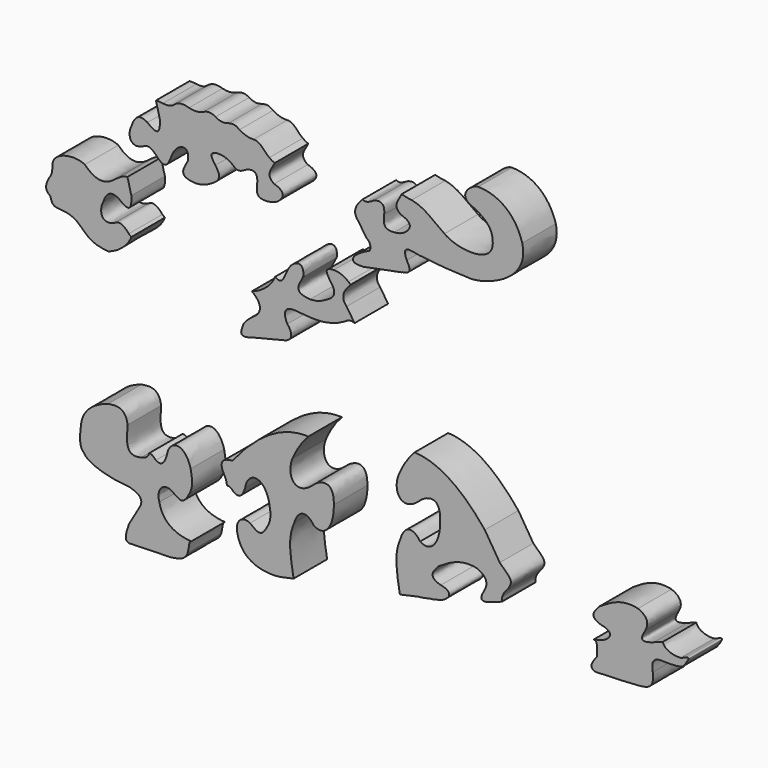
from build123d import *

# Parameters (mm, degrees)
F1_DEPTH = 12
F2_DEPTH = 12


# Not quite as in the source:
# - ends of sketch curves that miss each other by under 0.0002 mm in the source are joined


with BuildPart() as f1:
    # F0 (on Front) → F1 (new body)
    with BuildSketch(Plane.XZ):
        with BuildLine():
            add(Edge.make_bspline(
                [(-57.6632552731, -27.8370372235), (-56.8270192731, -27.7124932235), (-56.4328532731, -28.3077192235), (-55.7004402731, -28.9646112235)],
                knots=[0, 0, 0, 0, 1, 1, 1, 1], degree=3))
            add(Edge.make_bspline(
                [(-59.9392842731, -29.6536852235), (-58.5150639656, -29.3227779134), (-57.7620552726, -28.7312774051), (-57.6632552731, -27.8370372235)],
                knots=[0, 0, 0, 0, 0.574929609, 0.574929609, 0.574929609, 0.574929609], degree=3))
            add(Edge.make_bspline(
                [(-63.8231502731, -22.7211922235), (-63.9633372731, -26.5746232235), (-64.8168222731, -30.7897702235), (-59.9392842731, -29.6536852235)],
                knots=[0, 0, 0, 0, 1, 1, 1, 1], degree=3))
            add(Edge.make_bspline(
                [(-69.4192572731, -19.2131872235), (-67.9895642731, -18.9941012235), (-64.3453622731, -18.0729412235), (-63.8231502731, -22.7211922235)],
                knots=[0, 0, 0, 0, 1, 1, 1, 1], degree=3))
            add(Edge.make_bspline(
                [(-77.1869882731, -27.3985372235), (-76.9230312731, -23.4790862235), (-74.2488692731, -20.7941312235), (-69.4192572731, -19.2131872235)],
                knots=[0, 0, 0, 0, 1, 1, 1, 1], degree=3))
            add(Edge.make_bspline(
                [(-76.3099872731, -33.7881222235), (-77.6117482731, -32.8695732235), (-77.5381322731, -30.3005722235), (-77.1869882731, -27.3985372235)],
                knots=[0, 0, 0, 0, 1, 1, 1, 1], degree=3))
            add(Edge.make_bspline(
                [(-63.3637672731, -38.1313692235), (-70.7173222731, -37.7332332235), (-75.6068892731, -35.4201732235), (-76.3099872731, -33.7881222235)],
                knots=[0, 0, 0, 0, 1, 1, 1, 1], degree=3))
            add(Edge.make_bspline(
                [(-60.2316182731, -42.0569992235), (-58.8391352731, -39.2936542235), (-62.0487202731, -38.5416922235), (-63.3637672731, -38.1313692235)],
                knots=[0, 0, 0, 0, 1, 1, 1, 1], degree=3))
            Line((-60.2316182731, -42.0569992235), (-63.4055302731, -47.5278202235))
            add(Edge.make_bspline(
                [(-62.5285282731, -52.3304492235), (-65.2092132731, -52.7646142235), (-64.2890662731, -50.1306202235), (-63.4055302731, -47.5278202235)],
                knots=[0, 0, 0, 0, 1, 1, 1, 1], degree=3))
            Line((-62.5285282731, -52.3304492235), (-51.5033612731, -52.0381152235))
            add(Edge.make_bspline(
                [(-46.6172052731, -49.3653462235), (-47.5033612731, -51.7611842235), (-49.6774822731, -51.7306562235), (-51.5033612731, -52.0381152235)],
                knots=[0, 0, 0, 0, 1, 1, 1, 1], degree=3))
            add(Edge.make_bspline(
                [(-45.5744562731, -46.1050362235), (-46.3868670531, -46.3715316602), (-46.0201860134, -47.0933507408), (-46.6172052731, -49.3653462235)],
                knots=[0.3924968872, 0.3924968872, 0.3924968872, 0.3924968872, 1, 1, 1, 1], degree=3))
            add(Edge.make_bspline(
                [(-54.7190352731, -39.1963012235), (-53.7864772731, -43.8191412235), (-50.1763782731, -45.8004342235), (-45.5744562731, -46.1050362235)],
                knots=[0, 0, 0, 0, 1, 1, 1, 1], degree=3))
            add(Edge.make_bspline(
                [(-51.1901452731, -35.1662692235), (-53.7689652731, -33.8076662235), (-55.6370502731, -36.2625362235), (-54.7190352731, -39.1963012235)],
                knots=[0, 0, 0, 0, 1, 1, 1, 1], degree=3))
            add(Edge.make_bspline(
                [(-46.0534192731, -34.1222192235), (-47.9555772731, -37.9892172235), (-49.0004562731, -36.7478712235), (-51.1901452731, -35.1662692235)],
                knots=[0, 0, 0, 0, 1, 1, 1, 1], degree=3))
            add(Edge.make_bspline(
                [(-45.7610872731, -27.8788012235), (-45.3743582731, -29.9115232235), (-44.9107912731, -31.9365612235), (-46.0534192731, -34.1222192235)],
                knots=[0, 0, 0, 0, 1, 1, 1, 1], degree=3))
            add(Edge.make_bspline(
                [(-52.5682902731, -26.7094642235), (-51.8971942731, -22.2386062235), (-47.3982782731, -21.8283962235), (-45.7610872731, -27.8788012235)],
                knots=[0, 0, 0, 0, 1, 1, 1, 1], degree=3))
            add(Edge.make_bspline(
                [(-55.7004402731, -28.9646112235), (-53.8401442731, -30.1369062235), (-53.0759262731, -28.2868492235), (-52.5682902731, -26.7094642235)],
                knots=[0, 0, 0, 0, 1, 1, 1, 1], degree=3))
        make_face()
    extrude(amount=F1_DEPTH)


with BuildPart() as f1b:
    # F0 (on Front) → F1, piece 2 (new body)
    with BuildSketch(Plane.XZ):
        with BuildLine():
            add(Edge.make_bspline(
                [(-12.0773014723, -8.7989715469), (-14.2629566343, -11.097880595), (-15.5926600777, -13.4697155345), (-16.6487829582, -15.8648618052)],
                knots=[0.0115110713, 0.0115110713, 0.0115110713, 0.0115110713, 1, 1, 1, 1], degree=3))
            add(Edge.make_bspline(
                [(-33.8134335521, -21.9709454075), (-26.7640223709, -13.1322376429), (-19.5312883541, -8.4546031934), (-12.0773014723, -8.7989715469)],
                knots=[0, 0, 0, 0, 0.5332230593, 0.5332230593, 0.5332230593, 0.5332230593], degree=3))
            add(Edge.make_bspline(
                [(-36.1938665521, -26.1889054075), (-37.7022515521, -23.4593484075), (-36.7586165521, -22.1397024075), (-33.8134335521, -21.9709454075)],
                knots=[0, 0, 0, 0, 1, 1, 1, 1], degree=3))
            add(Edge.make_bspline(
                [(-36.1938665521, -26.1889054075), (-35.2106601216, -27.8341431077), (-35.7371349104, -28.0034519638), (-35.2542215521, -28.7155054075)],
                knots=[0, 0, 0, 0, 2.6956706561, 2.6956706561, 2.6956706561, 2.6956706561], degree=3))
            add(Edge.make_bspline(
                [(-35.2542215521, -28.7155054075), (-34.4179855521, -28.5909614075), (-34.0238195521, -29.1861874075), (-33.2914065521, -29.8430794075)],
                knots=[0, 0, 0, 0, 1, 1, 1, 1], degree=3))
            add(Edge.make_bspline(
                [(-33.2914065521, -29.8430794075), (-31.4311105521, -31.0153744075), (-30.6668925521, -29.1653174075), (-30.1592565521, -27.5879324075)],
                knots=[0, 0, 0, 0, 1, 1, 1, 1], degree=3))
            add(Edge.make_bspline(
                [(-30.1592565521, -27.5879324075), (-29.4881605521, -23.1170744075), (-24.9892445521, -22.7068644075), (-23.3520535521, -28.7572694075)],
                knots=[0, 0, 0, 0, 1, 1, 1, 1], degree=3))
            add(Edge.make_bspline(
                [(-23.3520535521, -28.7572694075), (-22.9653245521, -30.7899914075), (-22.5017575521, -32.8150294075), (-23.6443855521, -35.0006874075)],
                knots=[0, 0, 0, 0, 1, 1, 1, 1], degree=3))
            add(Edge.make_bspline(
                [(-23.6443855521, -35.0006874075), (-25.5465435521, -38.8676854075), (-26.5914225521, -37.6263394075), (-28.7811115521, -36.0447374075)],
                knots=[0, 0, 0, 0, 1, 1, 1, 1], degree=3))
            add(Edge.make_bspline(
                [(-28.7811115521, -36.0447374075), (-31.3599315521, -34.6861344075), (-33.2280165521, -37.1410044075), (-32.3100015521, -40.0747694075)],
                knots=[0, 0, 0, 0, 1, 1, 1, 1], degree=3))
            add(Edge.make_bspline(
                [(-32.3100015521, -40.0747694075), (-31.3655626309, -44.6390467683), (-27.808671917, -46.6098858118), (-23.2706547375, -46.9273209767)],
                knots=[0.0015526306, 0.0015526306, 0.0015526306, 0.0015526306, 0.9912302643, 0.9912302643, 0.9912302643, 0.9912302643], degree=3))
            add(Edge.make_bspline(
                [(-23.2706547375, -46.9273209767), (-23.2304424402, -46.9301338346), (-23.1901531038, -46.9328168656), (-23.1497878636, -46.9353707238)],
                knots=[0.9912302643, 0.9912302643, 0.9912302643, 0.9912302643, 1, 1, 1, 1], degree=3))
            add(Edge.make_bspline(
                [(-23.1497878636, -46.9353707238), (-21.813176476, -47.0200015094), (-20.6810826343, -46.9236295901), (-19.5101269181, -46.6634810166)],
                knots=[0.1098075094, 0.1098075094, 0.1098075094, 0.1098075094, 3.7697720097, 3.7697720097, 3.7697720097, 3.7697720097], degree=3))
            Line((-19.5101269181, -46.6634810166), (-16.2948955521, -45.9731464075))
            add(Edge.make_bspline(
                [(-16.1063455521, -31.8267744075), (-18.2630955521, -36.6973344075), (-17.0116295521, -41.3154354075), (-16.2948955521, -45.9731464075)],
                knots=[0, 0, 0, 0, 1, 1, 1, 1], degree=3))
            add(Edge.make_bspline(
                [(-10.5102365521, -30.7409634075), (-12.7108025521, -27.4498184075), (-15.1357915521, -28.4487944075), (-16.1063455521, -31.8267744075)],
                knots=[0, 0, 0, 0, 1, 1, 1, 1], degree=3))
            add(Edge.make_bspline(
                [(-4.7880627815, -23.6184258893), (-4.6595943077, -28.2050325034), (-6.7065542785, -33.0044090569), (-10.5102365521, -30.7409634075)],
                knots=[0.0038307729, 0.0038307729, 0.0038307729, 0.0038307729, 1, 1, 1, 1], degree=3))
            add(Edge.make_bspline(
                [(-10.2980750893, -20.2109066236), (-9.3285496951, -19.3834559666), (-4.7053523786, -16.6988469177), (-4.7880627815, -23.6184258893)],
                knots=[0, 0, 0, 0, 0.9989651443, 0.9989651443, 0.9989651443, 0.9989651443], degree=3))
            add(Edge.make_bspline(
                [(-16.6487829582, -15.8648618052), (-18.5621299308, -20.733127896), (-15.5459850899, -25.3383312754), (-10.2980750893, -20.2109066236)],
                knots=[0, 0, 0, 0, 0.9983595387, 0.9983595387, 0.9983595387, 0.9983595387], degree=3))
        make_face()
    extrude(amount=F1_DEPTH)


with BuildPart() as f1c:
    # F0 (on Front) → F1, piece 3 (new body)
    with BuildSketch(Plane.XZ):
        with BuildLine():
            add(Edge.make_bspline(
                [(23.548084, -38.2377454075), (22.7367236481, -38.1791038936), (21.4068074297, -38.7869122604), (19.444968, -38.9163794075)],
                knots=[0.5218030141, 0.5218030141, 0.5218030141, 0.5218030141, 1, 1, 1, 1], degree=3))
            add(Edge.make_bspline(
                [(23.548084, -38.2377454075), (24.992613, -37.9112934075), (26.754442, -37.5744944075), (27.651203, -36.5359454075)],
                knots=[0, 0, 0, 0, 1, 1, 1, 1], degree=3))
            add(Edge.make_bspline(
                [(27.651203, -36.5359454075), (29.183317, -35.1405314075), (27.428005, -34.1638224075), (25.813674, -33.9049404075)],
                knots=[0, 0, 0, 0, 1, 1, 1, 1], degree=3))
            add(Edge.make_bspline(
                [(25.813674, -33.9049404075), (22.067411, -32.7916104075), (23.602502, -31.0854724075), (25.187245, -29.3737634075)],
                knots=[0, 0, 0, 0, 1, 1, 1, 1], degree=3))
            add(Edge.make_bspline(
                [(25.187245, -29.3737634075), (28.494805, -27.1301704075), (31.936191, -25.3252374075), (36.233293, -26.3251364075)],
                knots=[0, 0, 0, 0, 1, 1, 1, 1], degree=3))
            add(Edge.make_bspline(
                [(36.233293, -26.3251364075), (38.786761, -27.3891544075), (39.546997, -28.9989354075), (38.258748, -31.2321714075)],
                knots=[0, 0, 0, 0, 1, 1, 1, 1], degree=3))
            add(Edge.make_bspline(
                [(38.258748, -31.2321714075), (37.095832, -33.2535824075), (36.489915, -34.9055584075), (40.701825, -33.3620344075)],
                knots=[0, 0, 0, 0, 1, 1, 1, 1], degree=3))
            Line((40.701825, -33.3620344075), (43.353712, -32.3806264075))
            Line((43.353712, -32.3806264075), (43.332833, -32.0674104075))
            add(Edge.make_bspline(
                [(44.37688, -29.3528814075), (43.463575, -30.5304284075), (43.186687, -31.5743714075), (43.332833, -32.0674104075)],
                knots=[0, 0, 0, 0, 1, 1, 1, 1], degree=3))
            add(Edge.make_bspline(
                [(42.706401, -22.7544864075), (45.116582, -25.3982344075), (47.511246, -25.9690594075), (44.37688, -29.3528814075)],
                knots=[0, 0, 0, 0, 1, 1, 1, 1], degree=3))
            Line((42.706401, -22.7544864075), (38.4217117968, -15.8964642394))
            add(Edge.make_bspline(
                [(18.3372880795, -2.9005945461), (24.854509263, -3.2016850576), (31.5408666488, -7.3418331273), (38.4217117968, -15.8964642394)],
                knots=[0.5332230593, 0.5332230593, 0.5332230593, 0.5332230593, 0.9994343196, 0.9994343196, 0.9994343196, 0.9994343196], degree=3))
            add(Edge.make_bspline(
                [(18.3372880798, -2.9005945469), (16.150032215, -5.2027873429), (14.8206613203, -7.5774711635), (13.765336, -9.9753144075)],
                knots=[0.0107004763, 0.0107004763, 0.0107004763, 0.0107004763, 1, 1, 1, 1], degree=3))
            add(Edge.make_bspline(
                [(13.765336, -9.9753144075), (11.863534, -14.8573274075), (14.90662, -19.4605244075), (20.154924, -14.2768024075)],
                knots=[0, 0, 0, 0, 1, 1, 1, 1], degree=3))
            add(Edge.make_bspline(
                [(20.154924, -14.2768024075), (21.124766, -13.4476894075), (25.754308, -10.7545304075), (25.667508, -17.7012834075)],
                knots=[0, 0, 0, 0, 1, 1, 1, 1], degree=3))
            add(Edge.make_bspline(
                [(25.667508, -17.7012834075), (25.785906, -22.3045624075), (23.709086, -27.1373974075), (19.904353, -24.8425864075)],
                knots=[0, 0, 0, 0, 1, 1, 1, 1], degree=3))
            add(Edge.make_bspline(
                [(19.904353, -24.8425864075), (17.703787, -21.5514414075), (15.278798, -22.5504174075), (14.308244, -25.9283974075)],
                knots=[0, 0, 0, 0, 1, 1, 1, 1], degree=3))
            add(Edge.make_bspline(
                [(14.308244, -25.9283974075), (12.151494, -30.7989574075), (13.40296, -35.4170584075), (14.119694, -40.0747694075)],
                knots=[0, 0, 0, 0, 1, 1, 1, 1], degree=3))
            Line((14.119694, -40.0747694075), (19.444968, -38.9163794075))
        make_face()
    extrude(amount=F1_DEPTH)


with BuildPart() as f1d:
    # F0 (on Front) → F1, piece 4 (new body)
    with BuildSketch(Plane.XZ):
        with BuildLine():
            add(Edge.make_bspline(
                [(69.5825900088, -33.375106762), (71.0271190088, -33.048654762), (72.7889480088, -32.711855762), (73.6857090088, -31.673306762)],
                knots=[0, 0, 0, 0, 1, 1, 1, 1], degree=3))
            add(Edge.make_bspline(
                [(70.5326770088, -37.436461762), (70.7388854588, -34.2937310778), (70.470917436, -33.4379439087), (69.5825900088, -33.375106762)],
                knots=[0, 0, 0, 0, 0.5225537589, 0.5225537589, 0.5225537589, 0.5225537589], degree=3))
            add(Edge.make_bspline(
                [(70.1985800088, -41.362091762), (67.8998800088, -40.913027762), (69.2521470088, -38.938115762), (70.5326770088, -37.436461762)],
                knots=[0, 0, 0, 0, 1, 1, 1, 1], degree=3))
            add(Edge.make_bspline(
                [(82.7271800088, -40.777422762), (76.0265000088, -41.297747762), (73.0870540088, -41.188363762), (70.1985800088, -41.362091762)],
                knots=[0, 0, 0, 0, 1, 1, 1, 1], degree=3))
            add(Edge.make_bspline(
                [(86.4857600088, -36.100077762), (87.0471980088, -40.271784762), (84.8822210088, -40.517448762), (82.7271800088, -40.777422762)],
                knots=[0, 0, 0, 0, 1, 1, 1, 1], degree=3))
            add(Edge.make_bspline(
                [(90.1608150088, -32.425022762), (86.0196750088, -32.014168762), (86.1514170088, -34.000296762), (86.4857600088, -36.100077762)],
                knots=[0, 0, 0, 0, 1, 1, 1, 1], degree=3))
            add(Edge.make_bspline(
                [(95.2557780088, -31.715069762), (94.4564490088, -32.435261762), (91.8822600088, -32.422067762), (90.1608150088, -32.425022762)],
                knots=[0, 0, 0, 0, 1, 1, 1, 1], degree=3))
            add(Edge.make_bspline(
                [(94.4205390088, -29.919303762), (95.4349870088, -29.763903762), (98.4317210088, -27.577872762), (95.2557780088, -31.715069762)],
                knots=[0, 0, 0, 0, 1, 1, 1, 1], degree=3))
            add(Edge.make_bspline(
                [(89.3882180088, -27.517987762), (89.6266837425, -29.1229862778), (92.2412113727, -30.0924736633), (94.4205390088, -29.919303762)],
                knots=[0.061437137, 0.061437137, 0.061437137, 0.061437137, 1, 1, 1, 1], degree=3))
            Line((89.3882180088, -27.517987762), (86.7363310088, -28.499395762))
            add(Edge.make_bspline(
                [(84.2932540088, -26.369532762), (83.1303380088, -28.390943762), (82.5244210088, -30.042919762), (86.7363310088, -28.499395762)],
                knots=[0, 0, 0, 0, 1, 1, 1, 1], degree=3))
            add(Edge.make_bspline(
                [(82.2677990088, -21.462497762), (84.8212670088, -22.526515762), (85.5815030088, -24.136296762), (84.2932540088, -26.369532762)],
                knots=[0, 0, 0, 0, 1, 1, 1, 1], degree=3))
            add(Edge.make_bspline(
                [(71.2217510088, -24.511124762), (74.5293110088, -22.267531762), (77.9706970088, -20.462598762), (82.2677990088, -21.462497762)],
                knots=[0, 0, 0, 0, 1, 1, 1, 1], degree=3))
            add(Edge.make_bspline(
                [(71.8481800088, -29.042301762), (68.1019170088, -27.928971762), (69.6370080088, -26.222833762), (71.2217510088, -24.511124762)],
                knots=[0, 0, 0, 0, 1, 1, 1, 1], degree=3))
            add(Edge.make_bspline(
                [(73.6857090088, -31.673306762), (75.2178230088, -30.277892762), (73.4625110088, -29.301183762), (71.8481800088, -29.042301762)],
                knots=[0, 0, 0, 0, 1, 1, 1, 1], degree=3))
        make_face()
    extrude(amount=F1_DEPTH)


with BuildPart() as f2:
    # F0 (on Front) → F2 (new body)
    with BuildSketch(Plane.XZ):
        with BuildLine():
            add(Edge.make_bspline(
                [(-69.3341766052, 19.2094726506), (-74.1750692719, 19.6497229208), (-75.1314553584, 21.0380042156), (-77.6239506052, 23.3082766506)],
                knots=[0.0007320493, 0.0007320493, 0.0007320493, 0.0007320493, 1, 1, 1, 1], degree=3))
            add(Edge.make_bspline(
                [(-69.3341766052, 19.2094726506), (-66.7822206052, 20.0185446506), (-63.8352736052, 22.0949326506), (-62.7357806052, 24.9935096506)],
                knots=[0, 0, 0, 0, 1, 1, 1, 1], degree=3))
            Line((-62.7357806052, 24.9935096506), (-63.4494586052, 25.5821016506))
            add(Edge.make_bspline(
                [(-67.4655646052, 27.0290806506), (-66.3722566052, 27.8827886506), (-65.0438666052, 27.4566046506), (-63.4494586052, 25.5821016506)],
                knots=[0, 0, 0, 0, 1, 1, 1, 1], degree=3))
            add(Edge.make_bspline(
                [(-70.7729466051, 31.2223666506), (-72.1112546052, 28.6972756506), (-71.3180636052, 25.2035596506), (-67.4655646052, 27.0290806506)],
                knots=[0, 0, 0, 0, 1, 1, 1, 1], degree=3))
            add(Edge.make_bspline(
                [(-66.2548266051, 33.4371306506), (-68.6348356051, 34.8837986506), (-69.9636576051, 33.7024986506), (-70.7729466051, 31.2223666506)],
                knots=[0, 0, 0, 0, 1, 1, 1, 1], degree=3))
            add(Edge.make_bspline(
                [(-62.7407346051, 35.4451836506), (-62.4579096051, 30.6639896506), (-64.2978666051, 31.8851406506), (-66.2548266051, 33.4371306506)],
                knots=[0, 0, 0, 0, 1, 1, 1, 1], degree=3))
            Line((-62.7407346052, 35.4451836506), (-63.8424736052, 39.7668176506))
            add(Edge.make_bspline(
                [(-67.2293236052, 38.1619616506), (-66.2370793141, 38.8034373603), (-65.4511063612, 39.6056437767), (-63.8424736052, 39.7668176506)],
                knots=[0, 0, 0, 0, 0.7472132911, 0.7472132911, 0.7472132911, 0.7472132911], degree=3))
            add(Edge.make_bspline(
                [(-76.0588506052, 38.9002166506), (-73.5317016052, 36.4139846506), (-70.7729876052, 35.1746446506), (-67.2293236052, 38.1619616506)],
                knots=[0, 0, 0, 0, 1, 1, 1, 1], degree=3))
            add(Edge.make_bspline(
                [(-85.3018006052, 36.0062576506), (-85.0422796052, 39.4741636506), (-78.7124016052, 40.4346446506), (-76.0588506052, 38.9002166506)],
                knots=[0, 0, 0, 0, 1, 1, 1, 1], degree=3))
            add(Edge.make_bspline(
                [(-86.1877056052, 32.3740446506), (-85.6062626052, 32.9607836506), (-85.2719136052, 34.0863706506), (-85.3018006052, 36.0062576506)],
                knots=[0, 0, 0, 0, 1, 1, 1, 1], degree=3))
            add(Edge.make_bspline(
                [(-85.8628736052, 27.7673336506), (-87.8424026052, 28.9089566506), (-87.1533056052, 30.6123946506), (-86.1877056052, 32.3740446506)],
                knots=[0, 0, 0, 0, 1, 1, 1, 1], degree=3))
            add(Edge.make_bspline(
                [(-83.4118676052, 25.3753876506), (-85.2312576052, 25.3612486506), (-85.6790836052, 26.4574196506), (-85.8628736052, 27.7673336506)],
                knots=[0, 0, 0, 0, 1, 1, 1, 1], degree=3))
            add(Edge.make_bspline(
                [(-77.6239506052, 23.3082766506), (-79.5033466052, 24.9955086506), (-81.4551646052, 25.2343016506), (-83.4118676052, 25.3753876506)],
                knots=[0, 0, 0, 0, 1, 1, 1, 1], degree=3))
        make_face()
    extrude(amount=F2_DEPTH)


with BuildPart() as f2b:
    # F0 (on Front) → F2, piece 2 (new body)
    with BuildSketch(Plane.XZ):
        with BuildLine():
            Line((-55.6936267021, 61.679005653), (-54.5918877021, 57.357371653))
            add(Edge.make_bspline(
                [(-54.5918877021, 57.357371653), (-54.3090627021, 52.576177653), (-56.1490197021, 53.797328653), (-58.1059797021, 55.349318653)],
                knots=[0, 0, 0, 0, 1, 1, 1, 1], degree=3))
            add(Edge.make_bspline(
                [(-58.1059797021, 55.349318653), (-60.4859887021, 56.795986653), (-61.8148107021, 55.614686653), (-62.6240997021, 53.134554653)],
                knots=[0, 0, 0, 0, 1, 1, 1, 1], degree=3))
            add(Edge.make_bspline(
                [(-62.6240997021, 53.134554653), (-63.9624077021, 50.609463653), (-63.1692167021, 47.115747653), (-59.3167177021, 48.941268653)],
                knots=[0, 0, 0, 0, 1, 1, 1, 1], degree=3))
            add(Edge.make_bspline(
                [(-59.3167177021, 48.941268653), (-58.2234097021, 49.794976653), (-56.8950197021, 49.368792653), (-55.3006117021, 47.494289653)],
                knots=[0, 0, 0, 0, 1, 1, 1, 1], degree=3))
            add(Edge.make_bspline(
                [(-55.3006117021, 47.494289653), (-52.2589077021, 44.482743653), (-51.9397537021, 47.963432653), (-50.9301437021, 49.797642653)],
                knots=[0, 0, 0, 0, 1, 1, 1, 1], degree=3))
            add(Edge.make_bspline(
                [(-50.9301437021, 49.797642653), (-49.7324007021, 52.682575653), (-45.9159127021, 53.956382653), (-46.5301467021, 49.502339653)],
                knots=[0, 0, 0, 0, 1, 1, 1, 1], degree=3))
            add(Edge.make_bspline(
                [(-46.5301467021, 49.502339653), (-47.8736427021, 47.033665653), (-49.5123127021, 44.815469653), (-44.5220927021, 44.511739653)],
                knots=[0, 0, 0, 0, 1, 1, 1, 1], degree=3))
            add(Edge.make_bspline(
                [(-44.5220927021, 44.511739653), (-42.2621227021, 44.496838653), (-40.6673497021, 45.403000653), (-39.1180677021, 46.372139653)],
                knots=[0, 0, 0, 0, 1, 1, 1, 1], degree=3))
            add(Edge.make_bspline(
                [(-39.1180677021, 46.372139653), (-36.8576087021, 47.834099653), (-37.5576867021, 49.343810653), (-38.7046437021, 50.860729653)],
                knots=[0, 0, 0, 0, 1, 1, 1, 1], degree=3))
            add(Edge.make_bspline(
                [(-38.7046437021, 50.860729653), (-39.7865937021, 52.463487653), (-40.8362027021, 54.054064653), (-37.7301467021, 54.079520653)],
                knots=[0, 0, 0, 0, 1, 1, 1, 1], degree=3))
            add(Edge.make_bspline(
                [(-37.7301467021, 54.079520653), (-36.4353057021, 54.059909653), (-35.0827527021, 53.722878653), (-33.5663897021, 52.484890653)],
                knots=[0, 0, 0, 0, 1, 1, 1, 1], degree=3))
            add(Edge.make_bspline(
                [(-33.5663897021, 52.484890653), (-32.1514467021, 51.031914653), (-30.9233427021, 52.070152653), (-29.6684077021, 52.750662653)],
                knots=[0, 0, 0, 0, 1, 1, 1, 1], degree=3))
            add(Edge.make_bspline(
                [(-29.6684077021, 52.750662653), (-27.4842107021, 53.532383653), (-26.5052297021, 52.688465653), (-26.7153867021, 50.240595653)],
                knots=[0, 0, 0, 0, 1, 1, 1, 1], degree=3))
            add(Edge.make_bspline(
                [(-26.7153867021, 50.240595653), (-26.6596527021, 48.588823653), (-27.6647707021, 46.399154653), (-23.8804897021, 46.637911653)],
                knots=[0, 0, 0, 0, 1, 1, 1, 1], degree=3))
            add(Edge.make_bspline(
                [(-23.8804897021, 46.637911653), (-22.0209217021, 46.765060653), (-20.9789237021, 47.371841653), (-20.2187437021, 48.143953653)],
                knots=[0, 0, 0, 0, 1, 1, 1, 1], degree=3))
            add(Edge.make_bspline(
                [(-20.2187437021, 48.143953653), (-18.2333017021, 50.109200653), (-20.2277467021, 51.191590653), (-21.8429047021, 51.658045653)],
                knots=[0, 0, 0, 0, 1, 1, 1, 1], degree=3))
            add(Edge.make_bspline(
                [(-21.8429047021, 51.658045653), (-23.4384897021, 52.654926653), (-23.4653657021, 53.838559653), (-22.7288117021, 55.113077653)],
                knots=[0, 0, 0, 0, 1, 1, 1, 1], degree=3))
            Line((-22.7288117021, 55.113077653), (-21.6934617021, 56.973479653))
            add(Edge.make_bspline(
                [(-23.2352727021, 57.856979653), (-22.7594168865, 57.4575588944), (-22.2313131482, 57.1792315199), (-21.6934617021, 56.973479653)],
                knots=[0, 0, 0, 0, 0.3520102972, 0.3520102972, 0.3520102972, 0.3520102972], degree=3))
            add(Edge.make_bspline(
                [(-27.7194147021, 60.960055653), (-25.7063097021, 61.042991653), (-24.8282167021, 58.869741653), (-23.2352727021, 57.856979653)],
                knots=[0, 0, 0, 0, 1, 1, 1, 1], degree=3))
            add(Edge.make_bspline(
                [(-31.8241107021, 62.052672653), (-30.6899077021, 61.532447653), (-29.7527837021, 60.880836653), (-27.7194147021, 60.960055653)],
                knots=[0, 0, 0, 0, 1, 1, 1, 1], degree=3))
            add(Edge.make_bspline(
                [(-34.8657187021, 62.731866653), (-33.9431007021, 62.815724653), (-33.1190787021, 63.234810653), (-31.8241107021, 62.052672653)],
                knots=[0, 0, 0, 0, 1, 1, 1, 1], degree=3))
            add(Edge.make_bspline(
                [(-38.5865247021, 63.115759653), (-37.5006467021, 62.370237653), (-36.2665627021, 62.217533653), (-34.8657187021, 62.731866653)],
                knots=[0, 0, 0, 0, 1, 1, 1, 1], degree=3))
            add(Edge.make_bspline(
                [(-42.0710857021, 63.233879653), (-40.8220077021, 63.894971653), (-39.6785477021, 63.711109653), (-38.5865247021, 63.115759653)],
                knots=[0, 0, 0, 0, 1, 1, 1, 1], degree=3))
            add(Edge.make_bspline(
                [(-46.2643717021, 62.909047653), (-44.8325377021, 62.574369653), (-43.4244627021, 62.548585653), (-42.0710857021, 63.233879653)],
                knots=[0, 0, 0, 0, 1, 1, 1, 1], degree=3))
            add(Edge.make_bspline(
                [(-50.2509497021, 62.525155653), (-49.2369337021, 63.212839653), (-47.9853327021, 63.478150653), (-46.2643717021, 62.909047653)],
                knots=[0, 0, 0, 0, 1, 1, 1, 1], degree=3))
            add(Edge.make_bspline(
                [(-53.7355117021, 61.580189653), (-52.6204677021, 61.500117653), (-51.5183507021, 61.310191653), (-50.2509497021, 62.525155653)],
                knots=[0, 0, 0, 0, 1, 1, 1, 1], degree=3))
            add(Edge.make_bspline(
                [(-55.6936267021, 61.679005653), (-55.1482861317, 61.730756549), (-54.5088903028, 61.7083162192), (-53.7355117021, 61.580189653)],
                knots=[0.7466347862, 0.7466347862, 0.7466347862, 0.7466347862, 1, 1, 1, 1], degree=3))
        make_face()
    extrude(amount=F2_DEPTH)


with BuildPart() as f2c:
    # F0 (on Front) → F2, piece 3 (new body)
    with BuildSketch(Plane.XZ):
        with BuildLine():
            add(Edge.make_bspline(
                [(1.140997, 24.057427), (0.4143117249, 24.4056286712), (-0.6256048198, 24.4537921928), (-1.31001, 23.762124)],
                knots=[0.3358339564, 0.3358339564, 0.3358339564, 0.3358339564, 0.7562493145, 0.7562493145, 0.7562493145, 0.7562493145], degree=3))
            add(Edge.make_bspline(
                [(1.140997, 24.057427), (0.10911, 25.489662), (-0.066584, 26.059833), (-1.132831, 27.512459)],
                knots=[0, 0, 0, 0, 1, 1, 1, 1], degree=3))
            add(Edge.make_bspline(
                [(-1.132831, 27.512459), (-2.46674, 28.924976), (-2.337564, 30.470498), (-1.073771, 32.119168)],
                knots=[0, 0, 0, 0, 1, 1, 1, 1], degree=3))
            Line((-1.073771, 32.119168), (0.048379, 33.418497))
            Line((0.048379, 33.418497), (-0.601285, 33.92051))
            add(Edge.make_bspline(
                [(-4.765042, 35.51514), (-3.470201, 35.495529), (-2.117648, 35.158498), (-0.601285, 33.92051)],
                knots=[0, 0, 0, 0, 1, 1, 1, 1], degree=3))
            add(Edge.make_bspline(
                [(-5.739539, 32.296349), (-6.821489, 33.899107), (-7.871098, 35.489684), (-4.765042, 35.51514)],
                knots=[0, 0, 0, 0, 1, 1, 1, 1], degree=3))
            add(Edge.make_bspline(
                [(-6.152963, 27.807759), (-3.892504, 29.269719), (-4.592582, 30.77943), (-5.739539, 32.296349)],
                knots=[0, 0, 0, 0, 1, 1, 1, 1], degree=3))
            add(Edge.make_bspline(
                [(-11.556988, 25.947359), (-9.297018, 25.932458), (-7.702245, 26.83862), (-6.152963, 27.807759)],
                knots=[0, 0, 0, 0, 1, 1, 1, 1], degree=3))
            add(Edge.make_bspline(
                [(-13.565042, 30.937959), (-14.908538, 28.469285), (-16.547208, 26.251089), (-11.556988, 25.947359)],
                knots=[0, 0, 0, 0, 1, 1, 1, 1], degree=3))
            add(Edge.make_bspline(
                [(-17.9579480355, 31.2268088923), (-16.7685376208, 34.1041335962), (-12.9807226228, 35.3846972885), (-13.565042, 30.937959)],
                knots=[0.0024980002, 0.0024980002, 0.0024980002, 0.0024980002, 1, 1, 1, 1], degree=3))
            add(Edge.make_bspline(
                [(-21.6147380355, 28.3348638923), (-19.3489549287, 26.5944978854), (-18.917449732, 29.5926467395), (-17.9579480355, 31.2268088923)],
                knots=[0.0948966859, 0.0948966859, 0.0948966859, 0.0948966859, 1, 1, 1, 1], degree=3))
            add(Edge.make_bspline(
                [(-28.2131340355, 22.5508268923), (-25.6611780355, 23.3598988923), (-22.7142310355, 25.4362868923), (-21.6147380355, 28.3348638923)],
                knots=[0, 0, 0, 0, 1, 1, 1, 1], degree=3))
            add(Edge.make_bspline(
                [(-26.824096, 17.029241), (-25.2017497424, 18.7885127325), (-25.8208700002, 20.6351262288), (-28.2131340355, 22.5508268923)],
                knots=[0, 0, 0, 0, 0.9999630963, 0.9999630963, 0.9999630963, 0.9999630963], degree=3))
            add(Edge.make_bspline(
                [(-30.603961, 13.603735), (-29.898478, 14.668907), (-28.313218, 16.035308), (-26.824096, 17.029241)],
                knots=[0, 0, 0, 0, 1, 1, 1, 1], degree=3))
            add(Edge.make_bspline(
                [(-28.212015, 10.916491), (-32.489368, 9.450163), (-31.269579, 11.724053), (-30.603961, 13.603735)],
                knots=[0, 0, 0, 0, 1, 1, 1, 1], degree=3))
            Line((-28.212015, 10.916491), (-18.777554, 13.255312))
            add(Edge.make_bspline(
                [(-18.08316, 17.590313), (-16.347829, 15.485903), (-16.73895, 13.78725), (-18.777554, 13.255312)],
                knots=[0, 0, 0, 0, 1, 1, 1, 1], degree=3))
            add(Edge.make_bspline(
                [(-15.1892, 21.69501), (-18.418522, 22.007017), (-19.730985, 20.896834), (-18.08316, 17.590313)],
                knots=[0, 0, 0, 0, 1, 1, 1, 1], degree=3))
            add(Edge.make_bspline(
                [(-1.31001, 23.762124), (-6.403165, 20.687442), (-10.785689, 21.244854), (-15.1892, 21.69501)],
                knots=[0, 0, 0, 0, 1, 1, 1, 1], degree=3))
        make_face()
    extrude(amount=F2_DEPTH)


with BuildPart() as f2d:
    # F0 (on Front) → F2, piece 4 (new body)
    with BuildSketch(Plane.XZ):
        with BuildLine():
            add(Edge.make_bspline(
                [(4.5253321359, 46.6179367231), (3.4934451359, 48.0501717231), (3.3177511359, 48.6203427231), (2.2515041359, 50.0729687231)],
                knots=[0, 0, 0, 0, 1, 1, 1, 1], degree=3))
            add(Edge.make_bspline(
                [(5.0864031359, 43.5172657231), (6.0313272824, 43.707837226), (5.8822401042, 45.9498901621), (4.5253321359, 46.6179367231)],
                knots=[0, 0, 0, 0, 0.6957238542, 0.6957238542, 0.6957238542, 0.6957238542], degree=3))
            add(Edge.make_bspline(
                [(1.1293571359, 41.0072007231), (2.2197231359, 42.0153747231), (3.5506401359, 42.8431377231), (5.0864031359, 43.5172657231)],
                knots=[0, 0, 0, 0, 1, 1, 1, 1], degree=3))
            add(Edge.make_bspline(
                [(3.6575911359, 39.0746357231), (1.2164261359, 38.9444357231), (-0.0140268641, 39.3193957231), (1.1293571359, 41.0072007231)],
                knots=[0, 0, 0, 0, 1, 1, 1, 1], degree=3))
            Line((3.6575911359, 39.0746357231), (14.5411301359, 41.2354057231))
            add(Edge.make_bspline(
                [(16.0960981359, 44.7596327231), (18.0703531359, 41.3189997231), (15.7572541359, 41.7824367231), (14.5411301359, 41.2354057231)],
                knots=[0, 0, 0, 0, 1, 1, 1, 1], degree=3))
            add(Edge.make_bspline(
                [(19.7038491359, 47.1790087231), (17.3362341359, 47.5033127231), (14.3880751359, 48.7373917231), (16.0960981359, 44.7596327231)],
                knots=[0, 0, 0, 0, 1, 1, 1, 1], degree=3))
            add(Edge.make_bspline(
                [(34.6461251359, 46.0568617231), (28.9467601359, 46.1229357231), (24.3276091359, 46.6519617231), (19.7038491359, 47.1790087231)],
                knots=[0, 0, 0, 0, 1, 1, 1, 1], degree=3))
            add(Edge.make_bspline(
                [(49.1454491359, 59.8474617231), (51.3903551359, 50.1800747231), (38.7751741359, 46.2719467231), (34.6461251359, 46.0568617231)],
                knots=[0, 0, 0, 0, 1, 1, 1, 1], degree=3))
            add(Edge.make_bspline(
                [(36.5655861359, 69.9172567231), (41.6036501359, 69.8747787231), (47.0213151359, 66.9937967231), (49.1454491359, 59.8474617231)],
                knots=[0, 0, 0, 0, 1, 1, 1, 1], degree=3))
            add(Edge.make_bspline(
                [(35.6206211359, 64.0998087231), (29.9587811359, 65.8704497231), (34.2366801359, 69.7204067231), (36.5655861359, 69.9172567231)],
                knots=[0, 0, 0, 0, 1, 1, 1, 1], degree=3))
            add(Edge.make_bspline(
                [(40.6702851359, 57.5736367231), (40.6831541359, 60.7384157231), (38.4164271359, 62.5734247231), (35.6206211359, 64.0998087231)],
                knots=[0, 0, 0, 0, 1, 1, 1, 1], degree=3))
            add(Edge.make_bspline(
                [(26.8796851359, 54.9749797231), (30.5509901359, 52.1310147231), (41.3247501359, 51.0854357231), (40.6702851359, 57.5736367231)],
                knots=[0, 0, 0, 0, 1, 1, 1, 1], degree=3))
            add(Edge.make_bspline(
                [(17.5040291359, 60.3942047231), (21.5489111359, 59.5401197231), (23.4462371359, 57.1484067231), (26.8796851359, 54.9749797231)],
                knots=[0, 0, 0, 0, 1, 1, 1, 1], degree=3))
            add(Edge.make_bspline(
                [(14.6559781359, 60.9696087231), (15.6328199859, 60.5993849706), (16.6559649971, 60.5055858935), (17.5040291359, 60.3942047231)],
                knots=[0.2599849916, 0.2599849916, 0.2599849916, 0.2599849916, 0.8890068216, 0.8890068216, 0.8890068216, 0.8890068216], degree=3))
            Line((14.6559781359, 60.9696087231), (13.6206281359, 59.1092067231))
            add(Edge.make_bspline(
                [(14.5065351359, 55.6541747231), (12.9109501359, 56.6510557231), (12.8840741359, 57.8346887231), (13.6206281359, 59.1092067231)],
                knots=[0, 0, 0, 0, 1, 1, 1, 1], degree=3))
            add(Edge.make_bspline(
                [(16.1306961359, 52.1400827231), (18.1161381359, 54.1053297231), (16.1216931359, 55.1877197231), (14.5065351359, 55.6541747231)],
                knots=[0, 0, 0, 0, 1, 1, 1, 1], degree=3))
            add(Edge.make_bspline(
                [(12.4689501359, 50.6340407231), (14.3285181359, 50.7611897231), (15.3705161359, 51.3679707231), (16.1306961359, 52.1400827231)],
                knots=[0, 0, 0, 0, 1, 1, 1, 1], degree=3))
            add(Edge.make_bspline(
                [(9.6340531359, 54.2367247231), (9.6897871359, 52.5849527231), (8.6846691359, 50.3952837231), (12.4689501359, 50.6340407231)],
                knots=[0, 0, 0, 0, 1, 1, 1, 1], degree=3))
            add(Edge.make_bspline(
                [(6.6810321359, 56.7467917231), (8.8652291359, 57.5285127231), (9.8442101359, 56.6845947231), (9.6340531359, 54.2367247231)],
                knots=[0, 0, 0, 0, 1, 1, 1, 1], degree=3))
            add(Edge.make_bspline(
                [(3.4327141359, 55.9790067231), (4.5796546959, 55.3496044179), (5.6211183549, 56.1754677706), (6.6810321359, 56.7467917231)],
                knots=[0.156546951, 0.156546951, 0.156546951, 0.156546951, 1, 1, 1, 1], degree=3))
            Line((3.4327141359, 55.9790067231), (2.3105641359, 54.6796777231))
            add(Edge.make_bspline(
                [(2.2515041359, 50.0729687231), (0.9175951359, 51.4854857231), (1.0467711359, 53.0310077231), (2.3105641359, 54.6796777231)],
                knots=[0, 0, 0, 0, 1, 1, 1, 1], degree=3))
        make_face()
    extrude(amount=F2_DEPTH)


solid = Compound([f1.part, f1b.part, f1c.part, f1d.part, f2.part, f2b.part, f2c.part, f2d.part])
